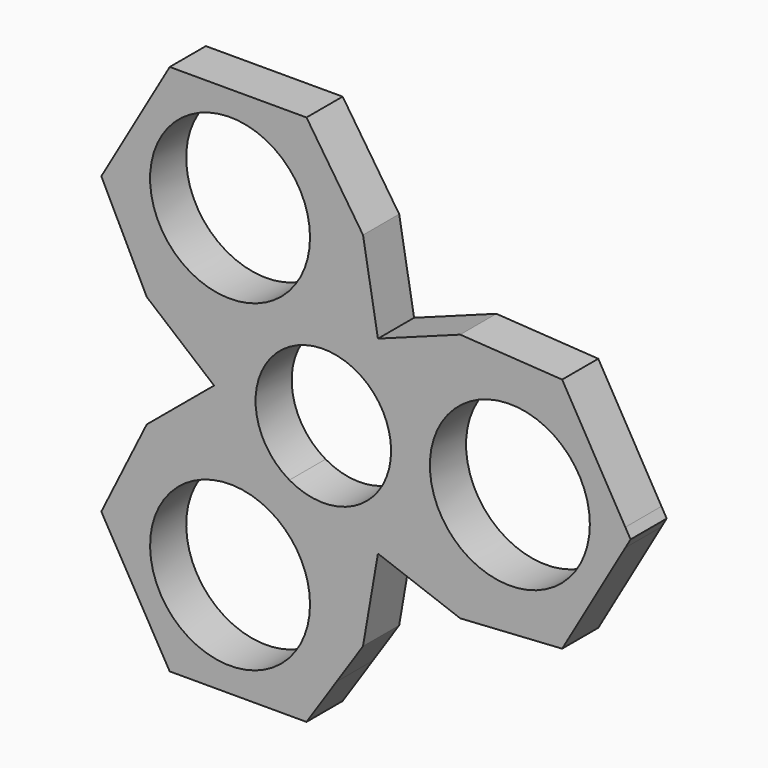
from build123d import *

# Parameters (mm, degrees)
F0_R     = 11.2395
F1_DEPTH = 6.35


# Not quite as in the source:
# - ends of sketch curves that miss each other by under 0.0002 mm in the source are joined


with BuildPart() as f1:
    # F0 (on Front) → F1 (new body)
    with BuildSketch(Plane.XZ):
        with BuildLine():
            Line((42.4467651581, 1.27), (33.5675281941, 16.6492895541))
            Line((33.5675281941, 16.6492895541), (19.2425445444, 17.5521669359))
            Line((19.2425445444, 17.5521669359), (7.6766035347, 13.2964561731))
            Line((7.6766035347, 13.2964561731), (5.579663063, 25.4405181745))
            Line((5.579663063, 25.4405181745), (-2.3645964913, 37.3949769354))
            Line((-2.3645964913, 37.3949769354), (-20.1235303163, 37.3949769354))
            ThreePointArc((-20.1235303163, 37.3949769354), (-21.3935303163, 37.054681461), (-22.3232348419, 36.1249769354))
            Line((-22.3232348419, 36.1249769354), (-31.2024718059, 20.7456873813))
            Line((-31.2024718059, 20.7456873813), (-31.1641125036, 20.668391129))
            Line((-31.1641125036, 20.668391129), (-27.8130050023, 13.9157122299))
            Line((-27.8130050023, 13.9157122299), (-24.8577417731, 7.960682843))
            Line((-24.8577417731, 7.960682843), (-24.8218947301, 7.8884489409))
            Line((-24.8218947301, 7.8884489409), (-15.353319828, -3.34766e-05))
            Line((-15.353319828, -3.34766e-05), (-24.8219665561, -7.8881291301))
            Line((-24.8219665561, -7.8881291301), (-24.8578663434, -7.9604670809))
            Line((-24.8578663434, -7.9604670809), (-31.1643564099, -20.6680233587))
            Line((-31.1643564099, -20.6680233587), (-31.2027017544, -20.7452890988))
            Line((-31.2027017544, -20.7452890988), (-22.3232348418, -36.1249769356))
            ThreePointArc((-22.3232348418, -36.1249769356), (-21.9195815404, -36.6510281597), (-21.3935303163, -37.0546814611))
            ThreePointArc((-21.3935303163, -37.0546814611), (-20.7809306909, -37.3084285342), (-20.1235303165, -37.3949769354))
            Line((-20.1235303165, -37.3949769354), (-2.3645964913, -37.3949769354))
            Line((-2.3645964913, -37.3949769354), (-2.3168550697, -37.3231360229))
            Line((-2.3168550697, -37.3231360229), (1.8552556307, -31.0449769354))
            Line((1.8552556307, -31.0449769354), (5.579663063, -25.4405181745))
            Line((5.579663063, -25.4405181745), (7.6765207659, -13.2964418818))
            Line((7.6765207659, -13.2964418818), (19.2425445444, -17.5521669359))
            Line((19.2425445444, -17.5521669359), (25.957862804, -17.1289127727))
            Line((25.957862804, -17.1289127727), (33.5675281941, -16.6492895541))
            Line((33.5675281941, -16.6492895541), (42.4467651581, -1.27))
            ThreePointArc((42.4467651581, -1.27), (42.7870606325, 0), (42.4467651581, 1.27))
        make_face()
        with BuildLine():
            ThreePointArc((-1.8702560234, -22.7067635073), (-22.8434485492, -28.3265135073), (-7.4900060234, -12.9730709815))
            ThreePointArc((-7.4900060234, -12.9730709815), (-3.3760634975, -17.0870135073), (-1.8702560234, -22.7067635073))
        make_face(mode=Mode.SUBTRACT)
        with BuildLine():
            ThreePointArc((-4.7625, -8.248891971), (-4.7625, 8.248891971), (9.525, 0))
            ThreePointArc((9.525, 0), (4.7625, -8.248891971), (-4.7625, -8.248891971))
        make_face(mode=Mode.SUBTRACT)
        with Locations((-13.1097560234, 22.7067635073)):
            Circle(F0_R, mode=Mode.SUBTRACT)
        with Locations((26.2195120463, 0.0001612286)):
            Circle(F0_R, mode=Mode.SUBTRACT)
        with BuildLine():
            Line((43.18, 0), (42.4467651581, 1.27))
            ThreePointArc((42.4467651581, 1.27), (42.7870606325, 0), (42.4467651581, -1.27))
            Line((42.4467651581, -1.27), (43.18, 0))
        make_face()
        with BuildLine():
            ThreePointArc((-22.3232348419, 36.1249769354), (-21.3935303163, 37.054681461), (-20.1235303163, 37.3949769354))
            Line((-20.1235303163, 37.3949769354), (-21.59, 37.3949769354))
            Line((-21.59, 37.3949769354), (-22.3232348419, 36.1249769354))
        make_face()
        with BuildLine():
            Line((-21.59, -37.3949769354), (-20.1235303165, -37.3949769354))
            ThreePointArc((-20.1235303165, -37.3949769354), (-20.7809306909, -37.3084285342), (-21.3935303163, -37.0546814611))
            Line((-21.3935303163, -37.0546814611), (-21.59, -37.3949769354))
        make_face()
        with BuildLine():
            Line((-21.59, -37.3949769354), (-21.3935303163, -37.0546814611))
            ThreePointArc((-21.3935303163, -37.0546814611), (-21.9195815404, -36.6510281597), (-22.3232348418, -36.1249769356))
            Line((-22.3232348418, -36.1249769356), (-21.59, -37.3949769354))
        make_face()
    extrude(amount=F1_DEPTH)


solid = f1.part
